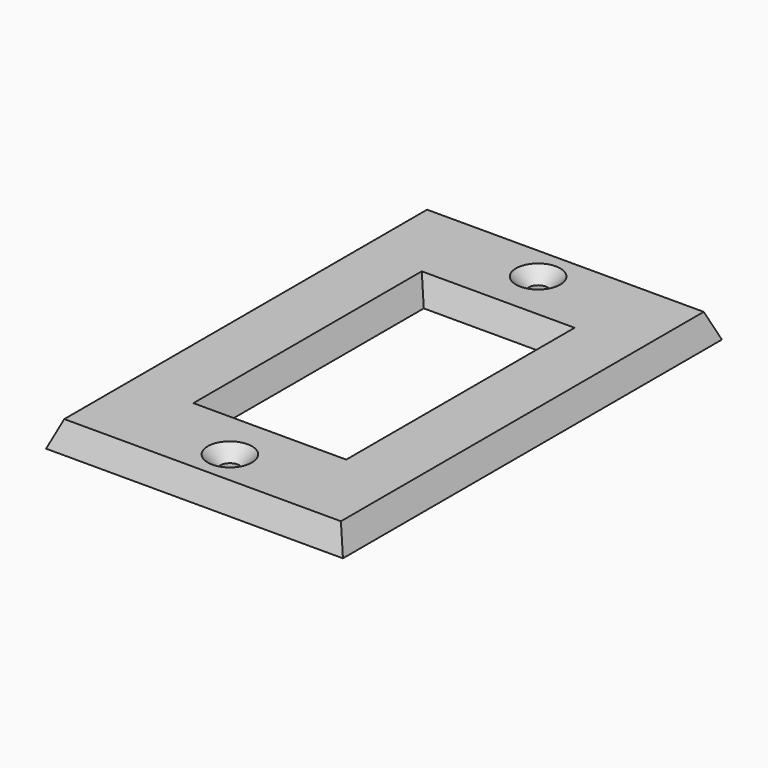
from build123d import *

# Parameters (mm, degrees)
F0_W     = 74.6125
F0_H     = 119.0625
F0_R     = 2.38125
F0_W_2   = 33.3375
F0_H_2   = 66.675
F1_DEPTH = 6.35
F2_SIZE2 = 6.34999
F2_SIZE  = 2.53999
F3_SIZE  = 3.175


# Not quite as in the source:
# - a fillet or chamfer is up to 0.001 mm smaller than in the source, because OpenCascade refuses the exact size


with BuildPart() as f1:
    # F0 (on Top) → F1 (new body)
    with BuildSketch(Plane.XY):
        Rectangle(F0_W, F0_H)
        with Locations((0, -48.41875)):
            Circle(F0_R, mode=Mode.SUBTRACT)
        Rectangle(F0_W_2, F0_H_2, mode=Mode.SUBTRACT)
        with Locations((0, 48.41875)):
            Circle(F0_R, mode=Mode.SUBTRACT)
    extrude(amount=F1_DEPTH)

    # F2 (size 2.54 and 6.35 in the source; OpenCascade refuses exactly that, so slightly less here)
    f2_edges = [f1.edges().sort_by_distance(p)[0] for p in [
        (-16.66875, 0, 6.35),
        (0, -33.3375, 6.35),
        (16.66875, 0, 6.35),
        (0, 33.3375, 6.35),
        (0, 59.53125, 6.35),
        (37.30625, 0, 6.35),
        (0, -59.53125, 6.35),
        (-37.30625, 0, 6.35),
    ]]
    f2_side = f1.faces().sort_by_distance((0, -58.126156, 6.35))[0]
    chamfer(f2_edges, length=F2_SIZE, length2=F2_SIZE2, reference=f2_side)

    # F3
    f3_edges = [f1.edges().sort_by_distance(p)[0] for p in [
        (-2.38125, -48.41875, 6.35),
        (-2.38125, 48.41875, 6.35),
    ]]
    chamfer(f3_edges, length=F3_SIZE)


solid = f1.part
